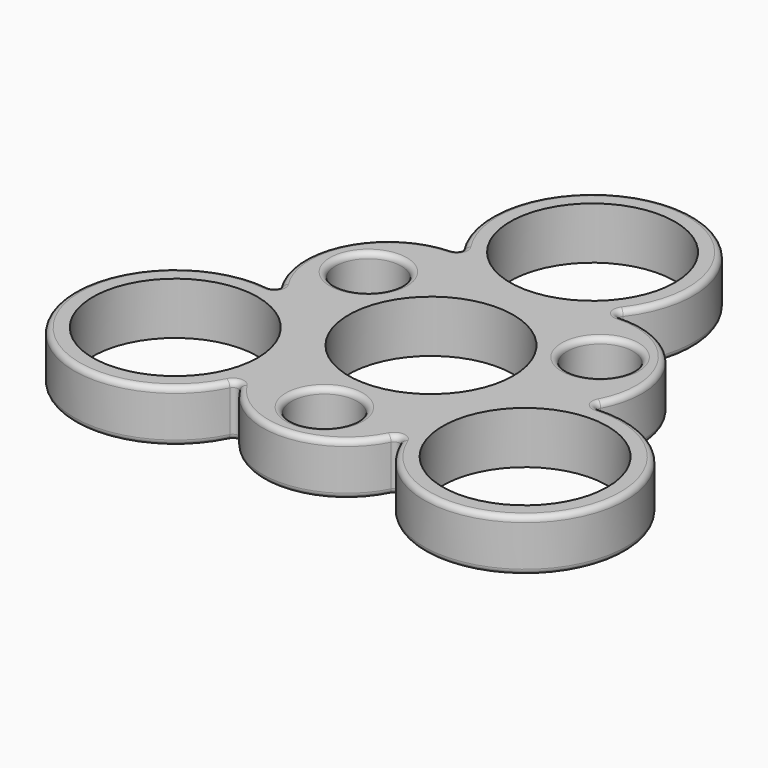
from build123d import *

# Parameters (mm, degrees)
F0_R     = 11.05
F0_R_2   = 4.4116454566
F1_DEPTH = 7
F2_R     = 0.75


with BuildPart() as f1:
    # F0 (on Top) → F1 (new body)
    with BuildSketch(Plane.XY):
        with BuildLine():
            ThreePointArc((21.1039623822, -0.1979522585), (21.3135291599, 12.6181340013), (9.3860647253, 17.3119147177))
            ThreePointArc((9.3860647253, 17.3119147177), (0.7280636191, 40.6149701394), (-10.3805495065, 18.3755436728))
            ThreePointArc((-10.3805495065, 18.3755436728), (-21.5785220669, 12.1461025902), (-19.6855902963, -0.5273868652))
            ThreePointArc((-19.6855902963, -0.5273868652), (-35.5376277242, -19.6769634799), (-10.7234128757, -18.1775914143))
            ThreePointArc((-10.7234128757, -18.1775914143), (0.2708600135, -24.7671246974), (10.2995255711, -16.7845278525))
            ThreePointArc((10.2995255711, -16.7845278525), (34.8095641051, -20.9380066594), (21.1039623822, -0.1979522585))
        make_face()
        with Locations((-23.4559034146, -13.5422721505)):
            Circle(F0_R, mode=Mode.SUBTRACT)
        with Locations((0.0371890647, -17.9136538016)):
            Circle(F0_R_2, mode=Mode.SUBTRACT)
        with Locations((23.4559034146, -13.5422721505)):
            Circle(F0_R, mode=Mode.SUBTRACT)
        Circle(F0_R, mode=Mode.SUBTRACT)
        with Locations((-15.5322737992, 8.924620226)):
            Circle(F0_R_2, mode=Mode.SUBTRACT)
        with Locations((15.4950847345, 8.9890335756)):
            Circle(F0_R_2, mode=Mode.SUBTRACT)
        with Locations((0, 27.084544301)):
            Circle(F0_R, mode=Mode.SUBTRACT)
    extrude(amount=F1_DEPTH)

    # F2
    f2_edges = [f1.edges().sort_by_distance(p)[0] for p in [
        (10.299526, -16.784528, 3.5),
        (21.103962, -0.197952, 3.5),
        (34.809564, -20.938007, 0),
        (34.809564, -20.938007, 7),
        (-19.68559, -0.527387, 3.5),
        (-10.723413, -18.177591, 3.5),
        (-35.537628, -19.676963, 0),
        (-35.537628, -19.676963, 7),
        (9.386065, 17.311915, 3.5),
        (-10.38055, 18.375544, 3.5),
        (0.728064, 40.61497, 0),
        (0.728064, 40.61497, 7),
        (-4.374456, -17.913654, 7),
        (4.448835, -17.913654, 3.5),
        (-4.374456, -17.913654, 0),
        (-11.120628, 8.92462, 3.5),
        (-19.943919, 8.92462, 0),
        (-19.943919, 8.92462, 7),
        (19.90673, 8.989034, 3.5),
        (11.083439, 8.989034, 0),
        (11.083439, 8.989034, 7),
        (21.313529, 12.618134, 0),
        (21.313529, 12.618134, 7),
        (-21.578522, 12.146103, 0),
        (-21.578522, 12.146103, 7),
        (0.27086, -24.767125, 0),
        (0.27086, -24.767125, 7),
    ]]
    fillet(f2_edges, radius=F2_R)


solid = f1.part
